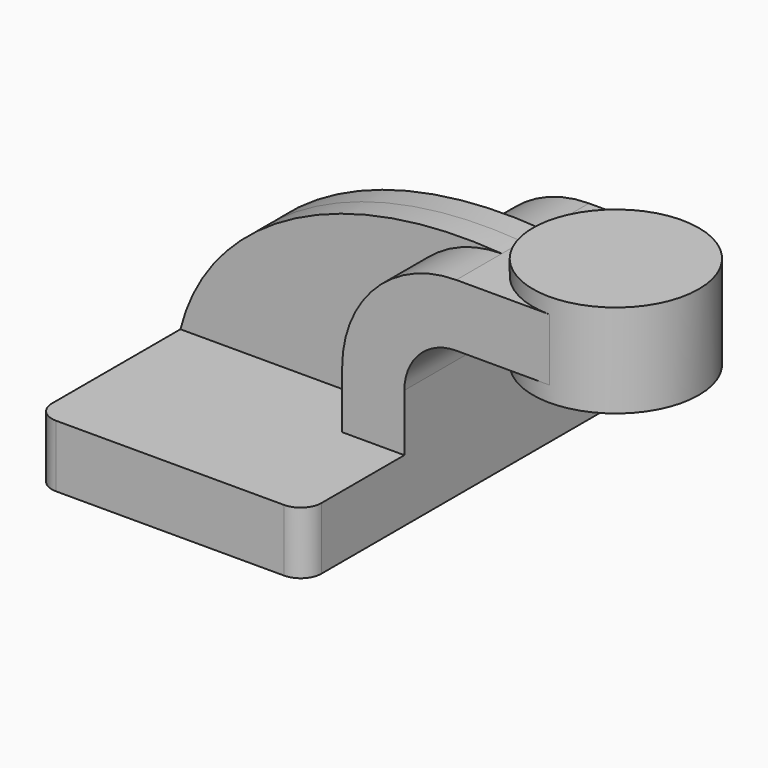
from build123d import *

# Parameters (mm, degrees)
F1_DEPTH = 63.5
F0_W     = 25.4
F0_H     = 19.05
F2_DEPTH = 25.4
F3_DEPTH = 7.9375
F5_R     = 6.35


# Not quite as in the source:
# - a feature names something its author has since deleted; it is built from what else it names


with BuildPart() as f1:
    # F0 (on Front) → F1 (new body, symmetric)
    with BuildSketch(Plane.XZ):
        Polygon((-41.275, 9.525), (-41.275, -9.525), (41.275, -9.525), (41.275, 9.525), (22.225, 9.525), align=None)
    extrude(amount=F1_DEPTH, both=True)

    # F0 (on Front) → F2 (join, symmetric)
    with BuildSketch(Plane.XZ):
        with BuildLine():
            Line((22.225, 9.525), (41.275, 9.525))
            Line((41.275, 9.525), (41.275, 27.0002))
            ThreePointArc((41.275, 27.0002), (45.9246798487, 38.2255201513), (57.15, 42.8752))
            Line((57.15, 42.8752), (60.325, 42.8752))
            Line((60.325, 42.8752), (60.325, 61.9252))
            Line((60.325, 61.9252), (57.15, 61.9252))
            ThreePointArc((57.15, 61.9252), (32.4542956671, 51.6959043329), (22.225, 27.0002))
            Line((22.225, 27.0002), (22.225, 9.525))
        make_face()
        with Locations((73.025, 52.4002)):
            Rectangle(F0_W, F0_H)
    extrude(amount=F2_DEPTH, both=True)

    # F0 (on Front) → F3 (join, symmetric)
    with BuildSketch(Plane.XZ):
        with BuildLine():
            add(Edge.make_bspline(
                [(-41.275, 9.525), (-33.0378338695, 42.7445545793), (5.4129776545, 65.891072154), (57.15, 61.9252)],
                knots=[0, 0, 0, 0, 111.5045361635, 111.5045361635, 111.5045361635, 111.5045361635], degree=3))
            Line((-41.275, 9.525), (22.225, 9.525))
            Line((22.225, 9.525), (22.225, 27.0002))
            ThreePointArc((22.225, 27.0002), (32.4542956671, 51.6959043329), (57.15, 61.9252))
        make_face()
    extrude(amount=F3_DEPTH, both=True)

    # F0 (on Front) → F4 (revolve)
    with BuildSketch(Plane.XZ):
        Polygon((85.725, 66.675), (85.725, 61.9252), (85.725, 42.8752), (85.725, 38.1), (111.125, 38.1), (111.125, 66.675), align=None)
    revolve(axis=Axis((85.725, 0, 52.3875), (0, 0, 1)))

    # F5
    f5_edges = [f1.edges().sort_by_distance(p)[0] for p in [
        (41.275, -63.5, 0),
        (-41.275, -63.5, 0),
        (41.275, 63.5, 0),
        (-41.275, 63.5, 0),
    ]]
    fillet(f5_edges, radius=F5_R)


solid = f1.part
